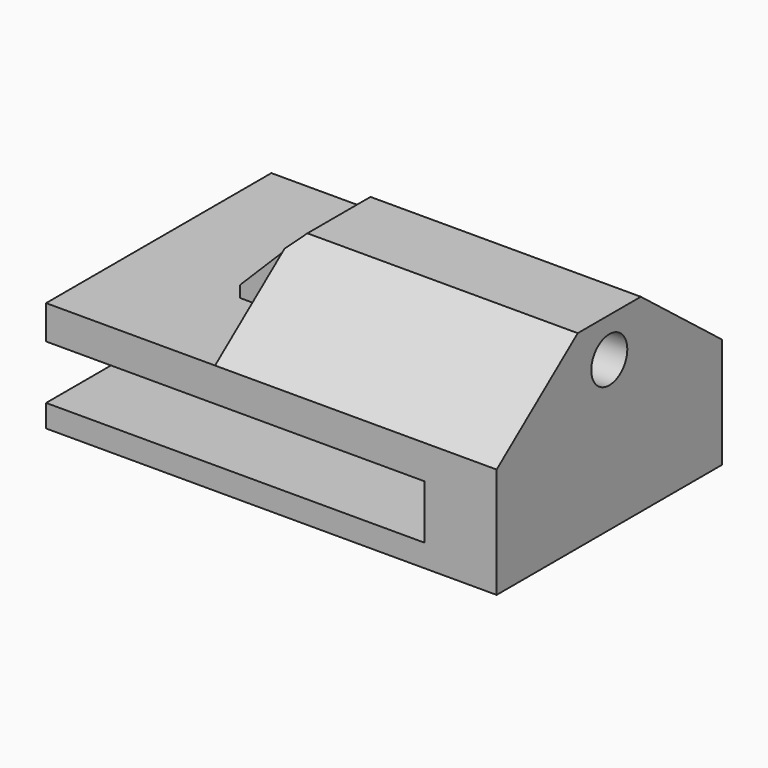
from build123d import *

# Parameters (mm, degrees)
F0_W        = 30
F0_H        = 7
F1_DEPTH    = 25
F2_W        = 30
F2_H        = 9
F3_DEPTH    = 7
F4_R        = 2
F5_DEPTH    = 25
F7_DEPTH    = 25
F8_T1_DEPTH = 37.8601958556


# Not quite as in the source:
# - a fillet or chamfer that OpenCascade refuses, or shapes differently, is made with other operations: its cross-section is extruded or revolved along the edge and cut away or added


with BuildPart() as f1:
    # F0 (on Front) → F1 (new body)
    with BuildSketch(Plane.XZ):
        Polygon((-40, 0), (0, 0), (0, 9.8), (-30, 9.8), (-40, 9.8), (-40, 6.8), (-6.3993203272, 6.8), (-6.3993203272, 2), (-40, 2), align=None)
        with Locations((-15, 13.3)):
            Rectangle(F0_W, F0_H)
    extrude(amount=F1_DEPTH)

    # F2 (on face) → F3 (cut)
    with BuildSketch(Plane.XY.offset(16.8)):
        with Locations((-15, -4.5)):
            Rectangle(F2_W, F2_H)
        with Locations((-15, -20.5)):
            Rectangle(F2_W, F2_H)
    extrude(amount=-F3_DEPTH, mode=Mode.SUBTRACT)

    # F4 (on face) → F5 (cut)
    with BuildSketch(Plane.YZ):
        with Locations((-12.5, 13.3)):
            Circle(F4_R)
    extrude(amount=-F5_DEPTH, mode=Mode.SUBTRACT)

    # F6 (on face) → F7 (join)
    with BuildSketch(Plane.YZ):
        Polygon((-16, 16.8), (-25, 9.8), (-16, 9.8), align=None)
        Polygon((0, 9.8), (-9, 16.8), (-9, 9.8), align=None)
    extrude(amount=-F7_DEPTH)

    # F8: chamfer of 6 on 1 edges, made by hand

    # F8_s2 → F8_t1 (cut)
    with BuildSketch(Plane.XZ.offset(-6.4300979278)):
        Polygon((-24, 16.8), (-30, 10.8), (-30, 16.8), align=None)
    extrude(amount=F8_T1_DEPTH, mode=Mode.SUBTRACT)


solid = f1.part
